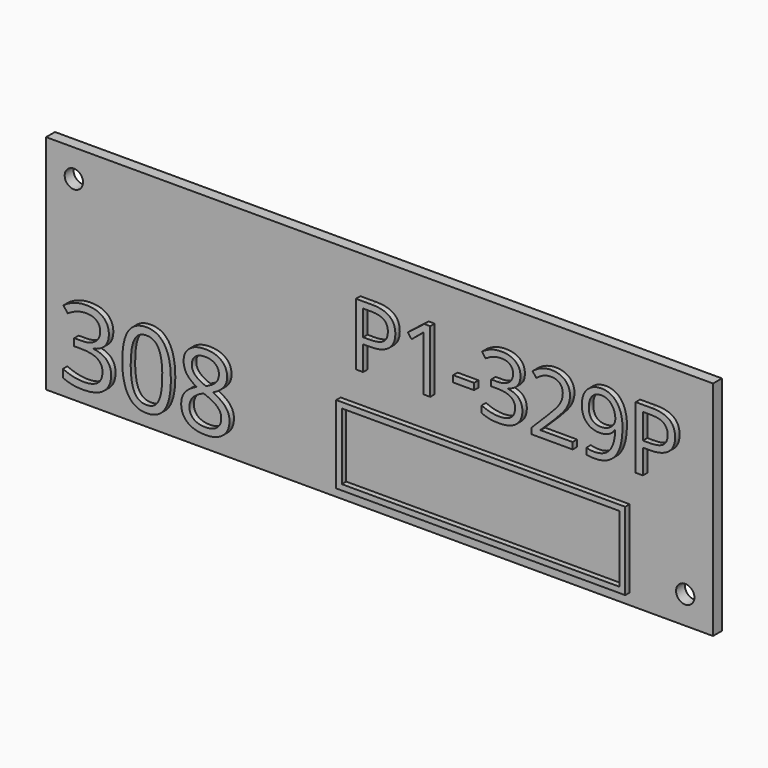
from build123d import *

# Parameters (mm, degrees)
F0_W         = 120
F0_H         = 40
F1_DEPTH     = 2
F3_D         = 3.3
F4_TEXT_SIZE = 15.681149951
F5_DEPTH     = 1
F6_TEXT_SIZE = 18.5155049272
F7_DEPTH     = 1
F8_W         = 52
F8_H         = 14
F8_W_2       = 49.99999962
F8_H_2       = 11.99999962
F9_DEPTH     = 1


# Not quite as in the source:
# - Text() gives the source's letters only with a copy of the font that has no kerning and outlines rounded to 1/6400 em; it was checked with that copy


with BuildPart() as f1:
    # F0 (on Front) → F1 (new body)
    with BuildSketch(Plane.XZ):
        Rectangle(F0_W, F0_H)
    extrude(amount=F1_DEPTH)

    # F3 (through all)
    with Locations(Plane.XZ.offset(2)):
        with Locations((-55, 15), (55, -15)):
            Hole(F3_D / 2)

    # F4 (on face) → F5 (join)
    with BuildSketch(Plane.XZ.offset(2)):
        with Locations((-5, 2)):
            Text('P1-329P', F4_TEXT_SIZE, font='Open Sans', text_align=(TextAlign.LEFT, TextAlign.BOTTOM))
    extrude(amount=F5_DEPTH)

    # F6 (on face) → F7 (join)
    with BuildSketch(Plane.XZ.offset(2)):
        with Locations((-57, -17)):
            Text('308', F6_TEXT_SIZE, font='Open Sans', text_align=(TextAlign.LEFT, TextAlign.BOTTOM))
    extrude(amount=F7_DEPTH)

    # F8 (on face) → F9 (join)
    with BuildSketch(Plane.XZ.offset(2)):
        with Locations((19, -11)):
            Rectangle(F8_W, F8_H)
        with Locations((19, -11)):
            Rectangle(F8_W_2, F8_H_2, mode=Mode.SUBTRACT)
    extrude(amount=F9_DEPTH)


solid = f1.part
